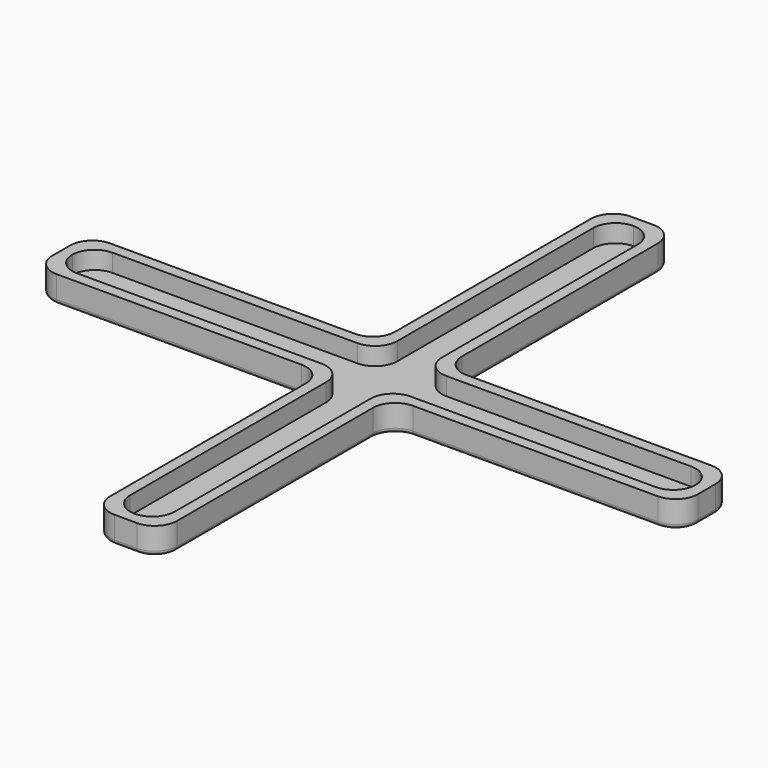
from build123d import *

# Parameters (mm, degrees)
F1_DEPTH = 2
F2_DEPTH = 6
F3_R     = 4.99999
F4_R     = 1


# Not quite as in the source:
# - a fillet or chamfer is up to 0.001 mm smaller than in the source, because OpenCascade refuses the exact size


with BuildPart() as f1:
    # F0 (on Top) → F1 (new body)
    with BuildSketch(Plane.XY):
        Polygon((5, 70), (0, 70), (-5, 70), (-5, 5), (-70, 5), (-70, -5), (-5, -5), (-5, -70), (0, -70), (5, -70), (5, -5), (70, -5), (70, 5), (5, 5), align=None)
    extrude(amount=F1_DEPTH)

    # F0 (on Top) → F2 (join)
    with BuildSketch(Plane.XY):
        Polygon((0, 72.5), (-7.5, 72.5), (-7.5, 7.5), (-72.5, 7.5), (-72.5, 6.8834697455), (-72.5, -7.5), (-7.5, -7.5), (-7.5, -72.5), (0, -72.5), (7.5, -72.5), (7.5, -7.5), (72.5, -7.5), (72.5, 7.5), (7.5, 7.5), (7.5, 72.5), align=None)
        Polygon((-5, 70), (0, 70), (5, 70), (5, 5), (70, 5), (70, -5), (5, -5), (5, -70), (0, -70), (-5, -70), (-5, -5), (-70, -5), (-70, 5), (-5, 5), align=None, mode=Mode.SUBTRACT)
    extrude(amount=F2_DEPTH)

    # F3 (radius 5 in the source; OpenCascade refuses exactly that, so slightly less here)
    f3_edges = [f1.edges().sort_by_distance(p)[0] for p in [
        (-5, 70, 4),
        (-70, 5, 4),
        (5, 70, 4),
        (70, 5, 4),
        (70, -5, 4),
        (5, -70, 4),
        (-70, -5, 4),
        (-5, -70, 4),
        (-7.5, 72.5, 3),
        (7.5, 72.5, 3),
        (72.5, 7.5, 3),
        (72.5, -7.5, 3),
        (7.5, -72.5, 3),
        (-72.5, 7.5, 3),
        (-72.5, -7.5, 3),
        (-7.5, -72.5, 3),
        (-7.5, -7.5, 3),
        (-5, 5, 4),
        (5, 5, 4),
        (5, -5, 4),
        (-7.5, 7.5, 3),
        (-5, -5, 4),
        (7.5, 7.5, 3),
        (7.5, -7.5, 3),
    ]]
    fillet(f3_edges, radius=F3_R)

    # F4
    f4_edges = [f1.edges().sort_by_distance(p)[0] for p in [
        (7.5, 40, 0),
    ]]
    fillet(f4_edges, radius=F4_R)


solid = f1.part
